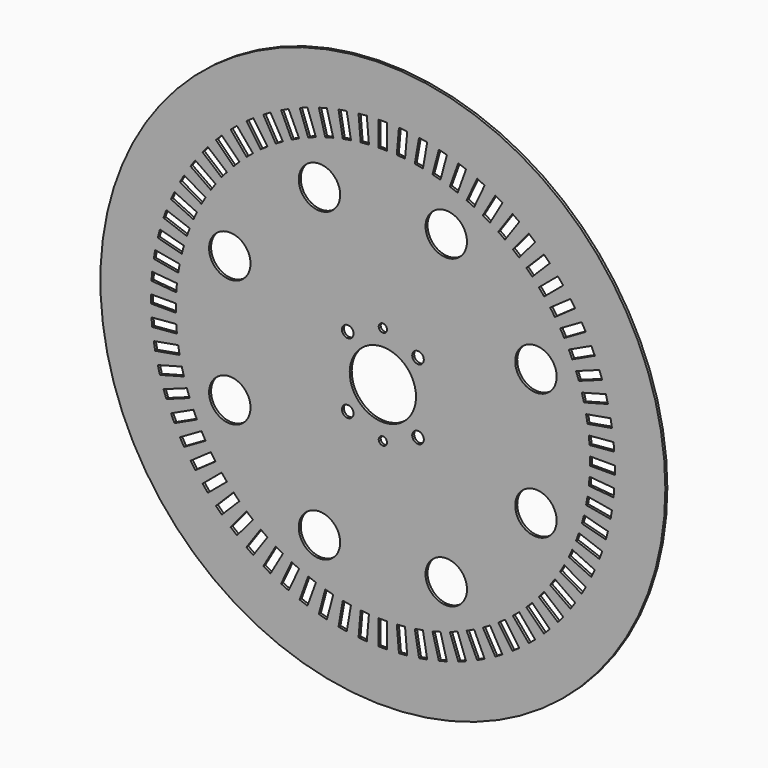
from build123d import *

# Parameters (mm, degrees)
F0_R     = 170.5
F1_DEPTH = 1.5
F3_DEPTH = 25
F5_DEPTH = 25
F7_DEPTH = 25


# Not quite as in the source:
# - ends of sketch curves that miss each other by under 0.0002 mm in the source are joined


with BuildPart() as f1:
    # F0 (on Front) → F1 (new body)
    with BuildSketch(Plane.XZ):
        Circle(F0_R)
        Polygon((-30, 0), (-15, 15), (0, 30), (30, 0), (15, -15), (0, -30), align=None, mode=Mode.SUBTRACT)
        with BuildLine():
            ThreePointArc((-14.1421356237, 14.1421356237), (7.6536686473, 18.4775906502), (20, 0))
            ThreePointArc((20, 0), (18.4775906502, -7.6536686473), (14.1421356237, -14.1421356237))
            Line((14.1421356237, -14.1421356237), (15, -15))
            Line((15, -15), (30, 0))
            Line((30, 0), (0, 30))
            Line((0, 30), (-15, 15))
            Line((-15, 15), (-14.1421356237, 14.1421356237))
        make_face()
        with BuildLine():
            ThreePointArc((14.1421356237, -14.1421356237), (-14.1421356237, -14.1421356237), (-14.1421356237, 14.1421356237))
            Line((-14.1421356237, 14.1421356237), (-15, 15))
            Line((-15, 15), (-30, 0))
            Line((-30, 0), (0, -30))
            Line((0, -30), (15, -15))
            Line((15, -15), (14.1421356237, -14.1421356237))
        make_face()
    extrude(amount=F1_DEPTH)

    # F2 (on face) → F3 (cut)
    with BuildSketch(Plane.XZ.offset(1.5)):
        with BuildLine():
            Line((-17.7132034356, 21.2132034356), (-21.2132034356, 21.2132034356))
            Line((-21.2132034356, 21.2132034356), (-21.2132034356, 17.7132034356))
            ThreePointArc((-21.2132034356, 17.7132034356), (-18.7383297014, 18.7383297014), (-17.7132034356, 21.2132034356))
        make_face()
        with BuildLine():
            ThreePointArc((-23.5394952244, 18.5981763778), (-22.4145176385, 19.9396439044), (-21.2132034356, 21.2132034356))
            ThreePointArc((-21.2132034356, 21.2132034356), (-19.9396439044, 22.4145176385), (-18.5981763778, 23.5394952244))
            ThreePointArc((-18.5981763778, 23.5394952244), (-23.6880771697, 23.6880771697), (-23.5394952244, 18.5981763778))
        make_face()
        with BuildLine():
            Line((-21.2132034356, 17.7132034356), (-21.2132034356, 21.2132034356))
            ThreePointArc((-21.2132034356, 21.2132034356), (-22.4145176385, 19.9396439044), (-23.5394952244, 18.5981763778))
            ThreePointArc((-23.5394952244, 18.5981763778), (-22.4576722575, 17.9419196889), (-21.2132034356, 17.7132034356))
        make_face()
        with BuildLine():
            ThreePointArc((-18.5981763778, 23.5394952244), (-19.9396439044, 22.4145176385), (-21.2132034356, 21.2132034356))
            Line((-21.2132034356, 21.2132034356), (-17.7132034356, 21.2132034356))
            ThreePointArc((-17.7132034356, 21.2132034356), (-17.9419196889, 22.4576722575), (-18.5981763778, 23.5394952244))
        make_face()
        with BuildLine():
            ThreePointArc((-21.2132034356, -21.2132034356), (-22.4145176385, -19.9396439044), (-23.5394952244, -18.5981763778))
            ThreePointArc((-23.5394952244, -18.5981763778), (-23.6880771697, -23.6880771697), (-18.5981763778, -23.5394952244))
            ThreePointArc((-18.5981763778, -23.5394952244), (-19.9396439044, -22.4145176385), (-21.2132034356, -21.2132034356))
        make_face()
        with BuildLine():
            Line((-21.2132034356, -21.2132034356), (-21.2132034356, -17.7132034356))
            ThreePointArc((-21.2132034356, -17.7132034356), (-22.4576722575, -17.9419196889), (-23.5394952244, -18.5981763778))
            ThreePointArc((-23.5394952244, -18.5981763778), (-22.4145176385, -19.9396439044), (-21.2132034356, -21.2132034356))
        make_face()
        with BuildLine():
            ThreePointArc((-17.7132034356, -21.2132034356), (-18.7383297014, -18.7383297014), (-21.2132034356, -17.7132034356))
            Line((-21.2132034356, -17.7132034356), (-21.2132034356, -21.2132034356))
            Line((-21.2132034356, -21.2132034356), (-17.7132034356, -21.2132034356))
        make_face()
        with BuildLine():
            Line((-17.7132034356, -21.2132034356), (-21.2132034356, -21.2132034356))
            ThreePointArc((-21.2132034356, -21.2132034356), (-19.9396439044, -22.4145176385), (-18.5981763778, -23.5394952244))
            ThreePointArc((-18.5981763778, -23.5394952244), (-17.9419196889, -22.4576722575), (-17.7132034356, -21.2132034356))
        make_face()
        with BuildLine():
            ThreePointArc((2.4978289184, -29.8958333333), (0, -27.5), (-2.4978289184, -29.8958333333))
            ThreePointArc((-2.4978289184, -29.8958333333), (0, -30), (2.4978289184, -29.8958333333))
        make_face()
        with BuildLine():
            ThreePointArc((2.4978289184, -29.8958333333), (0, -30), (-2.4978289184, -29.8958333333))
            ThreePointArc((-2.4978289184, -29.8958333333), (-0.0520946447, -32.4994571707), (2.5, -30))
            ThreePointArc((2.5, -30), (2.4994571707, -29.9479053553), (2.4978289184, -29.8958333333))
        make_face()
        with BuildLine():
            ThreePointArc((23.5394952244, -18.5981763778), (22.4145176385, -19.9396439044), (21.2132034356, -21.2132034356))
            ThreePointArc((21.2132034356, -21.2132034356), (19.9396439044, -22.4145176385), (18.5981763778, -23.5394952244))
            ThreePointArc((18.5981763778, -23.5394952244), (22.4576722575, -24.4844871823), (24.7132034356, -21.2132034356))
            ThreePointArc((24.7132034356, -21.2132034356), (24.406322699, -19.7800288581), (23.5394952244, -18.5981763778))
        make_face()
        with BuildLine():
            Line((21.2132034356, -21.2132034356), (21.2132034356, -17.7132034356))
            ThreePointArc((21.2132034356, -17.7132034356), (18.7383297014, -18.7383297014), (17.7132034356, -21.2132034356))
            Line((17.7132034356, -21.2132034356), (21.2132034356, -21.2132034356))
        make_face()
        with BuildLine():
            Line((21.2132034356, -21.2132034356), (17.7132034356, -21.2132034356))
            ThreePointArc((17.7132034356, -21.2132034356), (17.9419196889, -22.4576722575), (18.5981763778, -23.5394952244))
            ThreePointArc((18.5981763778, -23.5394952244), (19.9396439044, -22.4145176385), (21.2132034356, -21.2132034356))
        make_face()
        with BuildLine():
            ThreePointArc((23.5394952244, -18.5981763778), (22.4576722575, -17.9419196889), (21.2132034356, -17.7132034356))
            Line((21.2132034356, -17.7132034356), (21.2132034356, -21.2132034356))
            ThreePointArc((21.2132034356, -21.2132034356), (22.4145176385, -19.9396439044), (23.5394952244, -18.5981763778))
        make_face()
        with BuildLine():
            Line((21.2132034356, 21.2132034356), (17.7132034356, 21.2132034356))
            ThreePointArc((17.7132034356, 21.2132034356), (18.7383297014, 18.7383297014), (21.2132034356, 17.7132034356))
            Line((21.2132034356, 17.7132034356), (21.2132034356, 21.2132034356))
        make_face()
        with BuildLine():
            ThreePointArc((18.5981763778, 23.5394952244), (17.9419196889, 22.4576722575), (17.7132034356, 21.2132034356))
            Line((17.7132034356, 21.2132034356), (21.2132034356, 21.2132034356))
            ThreePointArc((21.2132034356, 21.2132034356), (19.9396439044, 22.4145176385), (18.5981763778, 23.5394952244))
        make_face()
        with BuildLine():
            ThreePointArc((23.5394952244, 18.5981763778), (22.4145176385, 19.9396439044), (21.2132034356, 21.2132034356))
            Line((21.2132034356, 21.2132034356), (21.2132034356, 17.7132034356))
            ThreePointArc((21.2132034356, 17.7132034356), (22.4576722575, 17.9419196889), (23.5394952244, 18.5981763778))
        make_face()
        with BuildLine():
            ThreePointArc((18.5981763778, 23.5394952244), (19.9396439044, 22.4145176385), (21.2132034356, 21.2132034356))
            ThreePointArc((21.2132034356, 21.2132034356), (22.4145176385, 19.9396439044), (23.5394952244, 18.5981763778))
            ThreePointArc((23.5394952244, 18.5981763778), (24.406322699, 19.7800288581), (24.7132034356, 21.2132034356))
            ThreePointArc((24.7132034356, 21.2132034356), (22.4576722575, 24.4844871823), (18.5981763778, 23.5394952244))
        make_face()
        with BuildLine():
            ThreePointArc((2.4978289184, 29.8958333333), (0, 30), (-2.4978289184, 29.8958333333))
            ThreePointArc((-2.4978289184, 29.8958333333), (0, 27.5), (2.4978289184, 29.8958333333))
        make_face()
        with BuildLine():
            ThreePointArc((2.5, 30), (-0.0520946447, 32.4994571707), (-2.4978289184, 29.8958333333))
            ThreePointArc((-2.4978289184, 29.8958333333), (0, 30), (2.4978289184, 29.8958333333))
            ThreePointArc((2.4978289184, 29.8958333333), (2.4994571707, 29.9479053553), (2.5, 30))
        make_face()
    extrude(amount=-F3_DEPTH, mode=Mode.SUBTRACT)

    # F4 (on face) → F5 (cut)
    with BuildSketch(Plane.XZ.offset(1.5)):
        with BuildLine():
            Line((-92.3879532511, 38.2683432365), (-92.3879532511, 25.7683432365))
            ThreePointArc((-92.3879532511, 25.7683432365), (-83.5491184863, 29.4295084717), (-79.8879532511, 38.2683432365))
            ThreePointArc((-79.8879532511, 38.2683432365), (-80.8394590947, 43.0518861411), (-83.5491184863, 47.1071780013))
            Line((-83.5491184863, 47.1071780013), (-92.3879532511, 38.2683432365))
        make_face()
        with BuildLine():
            ThreePointArc((-83.5491184863, 47.1071780013), (-103.9364474075, 43.0518861411), (-92.3879532511, 25.7683432365))
            Line((-92.3879532511, 25.7683432365), (-92.3879532511, 38.2683432365))
            Line((-92.3879532511, 38.2683432365), (-83.5491184863, 47.1071780013))
        make_face()
        with BuildLine():
            Line((-92.3879532511, -38.2683432365), (-83.5491184863, -47.1071780013))
            ThreePointArc((-83.5491184863, -47.1071780013), (-80.8394590947, -43.0518861411), (-79.8879532511, -38.2683432365))
            ThreePointArc((-79.8879532511, -38.2683432365), (-83.5491184863, -29.4295084717), (-92.3879532511, -25.7683432365))
            Line((-92.3879532511, -25.7683432365), (-92.3879532511, -38.2683432365))
        make_face()
        with BuildLine():
            ThreePointArc((-92.3879532511, -25.7683432365), (-103.9364474075, -43.0518861411), (-83.5491184863, -47.1071780013))
            Line((-83.5491184863, -47.1071780013), (-92.3879532511, -38.2683432365))
            Line((-92.3879532511, -38.2683432365), (-92.3879532511, -25.7683432365))
        make_face()
        with BuildLine():
            Line((-38.2683432365, -92.3879532511), (-25.7683432365, -92.3879532511))
            ThreePointArc((-25.7683432365, -92.3879532511), (-33.4848003319, -80.8394590947), (-47.1071780013, -83.5491184863))
            Line((-47.1071780013, -83.5491184863), (-38.2683432365, -92.3879532511))
        make_face()
        with BuildLine():
            ThreePointArc((-47.1071780013, -83.5491184863), (-43.0518861411, -103.9364474075), (-25.7683432365, -92.3879532511))
            Line((-25.7683432365, -92.3879532511), (-38.2683432365, -92.3879532511))
            Line((-38.2683432365, -92.3879532511), (-47.1071780013, -83.5491184863))
        make_face()
        with BuildLine():
            ThreePointArc((47.1071780013, -83.5491184863), (33.4848003319, -80.8394590947), (25.7683432365, -92.3879532511))
            Line((25.7683432365, -92.3879532511), (38.2683432365, -92.3879532511))
            Line((38.2683432365, -92.3879532511), (47.1071780013, -83.5491184863))
        make_face()
        with BuildLine():
            Line((38.2683432365, -92.3879532511), (25.7683432365, -92.3879532511))
            ThreePointArc((25.7683432365, -92.3879532511), (38.2683432365, -104.8879532511), (50.7683432365, -92.3879532511))
            ThreePointArc((50.7683432365, -92.3879532511), (49.8168373929, -87.6044103466), (47.1071780013, -83.5491184863))
            Line((47.1071780013, -83.5491184863), (38.2683432365, -92.3879532511))
        make_face()
        with BuildLine():
            ThreePointArc((92.3879532511, -25.7683432365), (80.8394590947, -33.4848003319), (83.5491184863, -47.1071780013))
            Line((83.5491184863, -47.1071780013), (92.3879532511, -38.2683432365))
            Line((92.3879532511, -38.2683432365), (92.3879532511, -25.7683432365))
        make_face()
        with BuildLine():
            Line((92.3879532511, -38.2683432365), (83.5491184863, -47.1071780013))
            ThreePointArc((83.5491184863, -47.1071780013), (97.1714961557, -49.8168373929), (104.8879532511, -38.2683432365))
            ThreePointArc((104.8879532511, -38.2683432365), (101.226788016, -29.4295084717), (92.3879532511, -25.7683432365))
            Line((92.3879532511, -25.7683432365), (92.3879532511, -38.2683432365))
        make_face()
        with BuildLine():
            ThreePointArc((83.5491184863, 47.1071780013), (80.8394590947, 33.4848003319), (92.3879532511, 25.7683432365))
            Line((92.3879532511, 25.7683432365), (92.3879532511, 38.2683432365))
            Line((92.3879532511, 38.2683432365), (83.5491184863, 47.1071780013))
        make_face()
        with BuildLine():
            Line((92.3879532511, 38.2683432365), (92.3879532511, 25.7683432365))
            ThreePointArc((92.3879532511, 25.7683432365), (101.226788016, 29.4295084717), (104.8879532511, 38.2683432365))
            ThreePointArc((104.8879532511, 38.2683432365), (97.1714961557, 49.8168373929), (83.5491184863, 47.1071780013))
            Line((83.5491184863, 47.1071780013), (92.3879532511, 38.2683432365))
        make_face()
        with BuildLine():
            ThreePointArc((25.7683432365, 92.3879532511), (33.4848003319, 80.8394590947), (47.1071780013, 83.5491184863))
            Line((47.1071780013, 83.5491184863), (38.2683432365, 92.3879532511))
            Line((38.2683432365, 92.3879532511), (25.7683432365, 92.3879532511))
        make_face()
        with BuildLine():
            Line((38.2683432365, 92.3879532511), (47.1071780013, 83.5491184863))
            ThreePointArc((47.1071780013, 83.5491184863), (49.8168373929, 87.6044103466), (50.7683432365, 92.3879532511))
            ThreePointArc((50.7683432365, 92.3879532511), (38.2683432365, 104.8879532511), (25.7683432365, 92.3879532511))
            Line((25.7683432365, 92.3879532511), (38.2683432365, 92.3879532511))
        make_face()
        with BuildLine():
            Line((-38.2683432365, 92.3879532511), (-47.1071780013, 83.5491184863))
            ThreePointArc((-47.1071780013, 83.5491184863), (-33.4848003319, 80.8394590947), (-25.7683432365, 92.3879532511))
            Line((-25.7683432365, 92.3879532511), (-38.2683432365, 92.3879532511))
        make_face()
        with BuildLine():
            ThreePointArc((-25.7683432365, 92.3879532511), (-43.0518861411, 103.9364474075), (-47.1071780013, 83.5491184863))
            Line((-47.1071780013, 83.5491184863), (-38.2683432365, 92.3879532511))
            Line((-38.2683432365, 92.3879532511), (-25.7683432365, 92.3879532511))
        make_face()
    extrude(amount=-F5_DEPTH, mode=Mode.SUBTRACT)

    # F6 (on face) → F7 (cut)
    with BuildSketch(Plane.XZ.offset(1.5)):
        with BuildLine():
            ThreePointArc((-2.49999995, 124.9749975005), (-6.24891e-05, 125), (2.4998749969, 124.975))
            Line((2.4998749969, 124.975), (2.4998749969, 139.975))
            Line((2.4998749969, 139.975), (-2.5, 139.975))
            Line((-2.5, 139.975), (-2.49999995, 124.9749975005))
        make_face()
        with BuildLine():
            ThreePointArc((8.4018020366, 124.7173192565), (10.8944055922, 124.5243427077), (13.3826511677, 124.2815539319))
            Line((13.3826511677, 124.2815539319), (14.6899873089, 139.2244744033))
            Line((14.6899873089, 139.2244744033), (9.7091383459, 139.6602422223))
            Line((9.7091383459, 139.6602422223), (8.4018020366, 124.7173192565))
        make_face()
        with BuildLine():
            ThreePointArc((19.2396612366, 123.5104669067), (21.7059606687, 123.1009799776), (24.1635772824, 122.6422501951))
            Line((24.1635772824, 122.6422501951), (26.7682999474, 137.4143664903))
            Line((26.7682999474, 137.4143664903), (21.8443842864, 138.2825856721))
            Line((21.8443842864, 138.2825856721), (19.2396612366, 123.5104669067))
        make_face()
        with BuildLine():
            ThreePointArc((29.9310949973, 121.363625326), (32.352320278, 120.7407444595), (34.7606039837, 120.0695648809))
            Line((34.7606039837, 120.0695648809), (38.6428896602, 134.5584522752))
            Line((38.6428896602, 134.5584522752), (33.8133812725, 135.8525151476))
            Line((33.8133812725, 135.8525151476), (29.9310949973, 121.363625326))
        make_face()
        with BuildLine():
            ThreePointArc((40.3947350523, 118.2931332752), (42.7524591952, 117.4615989707), (45.0930814996, 116.583077678))
            Line((45.0930814996, 116.583077678), (50.2233836495, 130.6784669898))
            Line((50.2233836495, 130.6784669898), (45.52503801, 132.3885249528))
            Line((45.52503801, 132.3885249528), (40.3947350523, 118.2931332752))
        make_face()
        with BuildLine():
            ThreePointArc((50.5509467824, 114.3223590528), (52.8272260833, 113.2884997886), (55.0823734373, 112.2093228592))
            Line((55.0823734373, 112.2093228592), (61.4216473634, 125.8039396647))
            Line((61.4216473634, 125.8039396647), (56.8902217196, 127.9169781448))
            Line((56.8902217196, 127.9169781448), (50.5509467824, 114.3223590528))
        make_face()
        with BuildLine():
            ThreePointArc((60.3224352841, 109.4815226483), (62.4999458829, 108.2532067176), (64.6524552536, 106.9815873395))
            Line((64.6524552536, 106.9815873395), (72.1524552536, 119.9719683963))
            Line((72.1524552536, 119.9719683963), (67.8224364905, 122.4719058947))
            Line((67.8224364905, 122.4719058947), (60.3224352841, 109.4815226483))
        make_face()
        with BuildLine():
            ThreePointArc((69.6348336296, 103.8074657497), (71.6970033558, 102.3940413784), (73.7304928471, 100.939657343))
            Line((73.7304928471, 100.939657343), (82.3341393924, 113.2269380073))
            Line((82.3341393924, 113.2269380073), (78.2384815675, 116.0947484902))
            Line((78.2384815675, 116.0947484902), (69.6348336296, 103.8074657497))
        make_face()
        with BuildLine():
            ThreePointArc((78.4172688444, 97.3433713561), (80.3484033414, 95.7555955571), (82.2473968704, 94.129515605))
            Line((82.2473968704, 94.129515605), (91.8892110157, 105.6201822518))
            Line((91.8892110157, 105.6201822518), (88.0590845581, 108.8340399498))
            Line((88.0590845581, 108.8340399498), (78.4172688444, 97.3433713561))
        make_face()
        with BuildLine():
            ThreePointArc((86.6029012938, 90.138435129), (88.3883034619, 88.3883918347), (90.1383485412, 86.6029914164))
            Line((90.1383485412, 86.6029914164), (100.744950259, 97.2095931342))
            Line((100.744950259, 97.2095931342), (97.2095047436, 100.7450386496))
            Line((97.2095047436, 100.7450386496), (86.6029012938, 90.138435129))
        make_face()
        with BuildLine():
            ThreePointArc((94.129433372, 82.2474909834), (95.7555152227, 80.3484990802), (97.3432929526, 78.4173661707))
            Line((97.3432929526, 78.4173661707), (108.8339595993, 88.059180316))
            Line((108.8339595993, 88.059180316), (105.6201019014, 91.8893067737))
            Line((105.6201019014, 91.8893067737), (94.129433372, 82.2474909834))
        make_face()
        with BuildLine():
            ThreePointArc((100.9395836253, 73.7305937691), (102.3939696939, 71.6971057319), (103.807396127, 69.6349374188))
            Line((103.807396127, 69.6349374188), (116.0946767914, 78.2385839641))
            Line((116.0946767914, 78.2385839641), (113.2268663085, 82.334241789))
            Line((113.2268663085, 82.334241789), (100.9395836253, 73.7305937691))
        make_face()
        with BuildLine():
            ThreePointArc((106.9815226983, 64.6525622164), (108.2531442285, 62.5000541171), (109.4814623364, 60.3225447464))
            Line((109.4814623364, 60.3225447464), (122.4718433932, 67.8225447464))
            Line((122.4718433932, 67.8225447464), (119.9719058947, 72.1525635095))
            Line((119.9719058947, 72.1525635095), (106.9815226983, 64.6525622164))
        make_face()
        with BuildLine():
            ThreePointArc((112.2092677864, 55.082485627), (113.2884469705, 52.8273393519), (114.3223085107, 50.5510610848))
            Line((114.3223085107, 50.5510610848), (127.9169253162, 56.8903350109))
            Line((127.9169253162, 56.8903350109), (125.8038868361, 61.4217606547))
            Line((125.8038868361, 61.4217606547), (112.2092677864, 55.082485627))
        make_face()
        with BuildLine():
            ThreePointArc((116.5830325927, 45.0931980622), (117.4615562257, 42.7525766362), (118.2930928874, 40.3948533247))
            Line((118.2930928874, 40.3948533247), (132.3884821992, 45.5251554746))
            Line((132.3884821992, 45.5251554746), (130.6784242362, 50.223501114))
            Line((130.6784242362, 50.223501114), (116.5830325927, 45.0931980622))
        make_face()
        with BuildLine():
            ThreePointArc((120.0695301263, 34.7607240322), (120.7407121128, 32.3524409976), (121.3635954, 29.9312163397))
            Line((121.3635954, 29.9312163397), (135.8524827944, 33.8135020162))
            Line((135.8524827944, 33.8135020162), (134.5584199221, 38.6430104039))
            Line((134.5584199221, 38.6430104039), (120.0695301263, 34.7607240322))
        make_face()
        with BuildLine():
            ThreePointArc((122.6422260357, 24.1636999032), (123.1009582754, 21.7060837481), (123.5104476703, 19.2397847254))
            Line((123.5104476703, 19.2397847254), (138.2825639655, 21.8445073904))
            Line((138.2825639655, 21.8445073904), (137.4143447837, 26.7684230515))
            Line((137.4143447837, 26.7684230515), (122.6422260357, 24.1636999032))
        make_face()
        with BuildLine():
            ThreePointArc((124.2815405515, 13.3827754275), (124.5243318152, 10.8945300947), (124.7173108561, 8.4019267321))
            Line((124.7173108561, 8.4019267321), (139.6602313275, 9.7092628733))
            Line((139.6602313275, 9.7092628733), (139.2244635085, 14.6901118363))
            Line((139.2244635085, 14.6901118363), (124.2815405515, 13.3827754275))
        make_face()
        with BuildLine():
            ThreePointArc((124.9749975005, 2.49999995), (124.9937492188, 1.2500624859), (125, 0))
            ThreePointArc((125, 0), (124.9937498437, -1.25), (124.975, -2.4998749969))
            Line((124.975, -2.4998749969), (139.975, -2.4998749969))
            Line((139.975, -2.4998749969), (139.975, 2.5))
            Line((139.975, 2.5), (124.9749975005, 2.49999995))
        make_face()
        with BuildLine():
            Line((139.6602422223, -9.7091383459), (124.7173217509, -8.4018022047))
            ThreePointArc((124.7173217509, -8.4018022047), (124.5243427077, -10.8944055922), (124.2815539319, -13.3826511677))
            Line((124.2815539319, -13.3826511677), (139.2244744033, -14.6899873089))
            Line((139.2244744033, -14.6899873089), (139.6602422223, -9.7091383459))
        make_face()
        with BuildLine():
            Line((138.2825856721, -21.8443842864), (123.5104693769, -19.2396616214))
            ThreePointArc((123.5104693769, -19.2396616214), (123.1009799776, -21.7059606687), (122.6422501951, -24.1635772824))
            Line((122.6422501951, -24.1635772824), (137.4143664903, -26.7682999474))
            Line((137.4143664903, -26.7682999474), (138.2825856721, -21.8443842864))
        make_face()
        with BuildLine():
            Line((135.8525151476, -33.8133812725), (121.3636277532, -29.931095596))
            ThreePointArc((121.3636277532, -29.931095596), (120.7407444595, -32.352320278), (120.0695648809, -34.7606039837))
            Line((120.0695648809, -34.7606039837), (134.5584522752, -38.6428896602))
            Line((134.5584522752, -38.6428896602), (135.8525151476, -33.8133812725))
        make_face()
        with BuildLine():
            Line((127.9169781448, -56.8902217196), (114.3223613393, -50.5509477935))
            ThreePointArc((114.3223613393, -50.5509477935), (113.2884997886, -52.8272260833), (112.2093228592, -55.0823734373))
            Line((112.2093228592, -55.0823734373), (125.8039396647, -61.4216473634))
            Line((125.8039396647, -61.4216473634), (127.9169781448, -56.8902217196))
        make_face()
        with BuildLine():
            Line((132.3885249528, -45.52503801), (118.293135641, -40.3947358602))
            ThreePointArc((118.293135641, -40.3947358602), (117.4615989707, -42.7524591952), (116.583077678, -45.0930814996))
            Line((116.583077678, -45.0930814996), (130.6784669898, -50.2233836495))
            Line((130.6784669898, -50.2233836495), (132.3885249528, -45.52503801))
        make_face()
        with BuildLine():
            Line((122.4719058947, -67.8224364905), (109.481524838, -60.3224364905))
            ThreePointArc((109.481524838, -60.3224364905), (108.2532067176, -62.4999458829), (106.9815873395, -64.6524552536))
            Line((106.9815873395, -64.6524552536), (119.9719683963, -72.1524552536))
            Line((119.9719683963, -72.1524552536), (122.4719058947, -67.8224364905))
        make_face()
        with BuildLine():
            Line((116.0947484902, -78.2384815675), (103.8074678259, -69.6348350222))
            ThreePointArc((103.8074678259, -69.6348350222), (102.3940413784, -71.6970033558), (100.939657343, -73.7304928471))
            Line((100.939657343, -73.7304928471), (113.2269380073, -82.3341393924))
            Line((113.2269380073, -82.3341393924), (116.0947484902, -78.2384815675))
        make_face()
        with BuildLine():
            Line((108.8340399498, -88.0590845581), (97.343373303, -78.4172704128))
            ThreePointArc((97.343373303, -78.4172704128), (95.7555955571, -80.3484033414), (94.129515605, -82.2473968704))
            Line((94.129515605, -82.2473968704), (105.6201822518, -91.8892110157))
            Line((105.6201822518, -91.8892110157), (108.8340399498, -88.0590845581))
        make_face()
        with BuildLine():
            Line((100.7450386496, -97.2095047436), (90.1384369318, -86.6029030258))
            ThreePointArc((90.1384369318, -86.6029030258), (88.3883918347, -88.3883034619), (86.6029914164, -90.1383485412))
            Line((86.6029914164, -90.1383485412), (97.2095931342, -100.744950259))
            Line((97.2095931342, -100.744950259), (100.7450386496, -97.2095047436))
        make_face()
        with BuildLine():
            Line((91.8893067737, -105.6201019014), (82.2474926284, -94.1294352546))
            ThreePointArc((82.2474926284, -94.1294352546), (80.3484990802, -95.7555152227), (78.4173661707, -97.3432929526))
            Line((78.4173661707, -97.3432929526), (88.059180316, -108.8339595993))
            Line((88.059180316, -108.8339595993), (91.8893067737, -105.6201019014))
        make_face()
        with BuildLine():
            Line((82.334241789, -113.2268663085), (73.7305952437, -100.9395856441))
            ThreePointArc((73.7305952437, -100.9395856441), (71.6971057319, -102.3939696939), (69.6349374188, -103.807396127))
            Line((69.6349374188, -103.807396127), (78.2385839641, -116.0946767914))
            Line((78.2385839641, -116.0946767914), (82.334241789, -113.2268663085))
        make_face()
        with BuildLine():
            Line((72.1525635095, -119.9719058947), (64.6525635095, -106.981524838))
            ThreePointArc((64.6525635095, -106.981524838), (62.5000541171, -108.2531442285), (60.3225447464, -109.4814623364))
            Line((60.3225447464, -109.4814623364), (67.8225447464, -122.4718433932))
            Line((67.8225447464, -122.4718433932), (72.1525635095, -119.9719058947))
        make_face()
        with BuildLine():
            Line((50.223501114, -130.6784242362), (45.0931989641, -116.5830349244))
            ThreePointArc((45.0931989641, -116.5830349244), (42.7525766362, -117.4615562257), (40.3948533247, -118.2930928874))
            Line((40.3948533247, -118.2930928874), (45.5251554746, -132.3884821992))
            Line((45.5251554746, -132.3884821992), (50.223501114, -130.6784242362))
        make_face()
        with BuildLine():
            Line((38.6430104039, -134.5584199221), (34.7607247274, -120.0695325277))
            ThreePointArc((34.7607247274, -120.0695325277), (32.3524409976, -120.7407121128), (29.9312163397, -121.3635954))
            Line((29.9312163397, -121.3635954), (33.8135020162, -135.8524827944))
            Line((33.8135020162, -135.8524827944), (38.6430104039, -134.5584199221))
        make_face()
        with BuildLine():
            Line((26.7684230515, -137.4143447837), (24.1637003865, -122.6422284885))
            ThreePointArc((24.1637003865, -122.6422284885), (21.7060837481, -123.1009582754), (19.2397847254, -123.5104476703))
            Line((19.2397847254, -123.5104476703), (21.8445073904, -138.2825639655))
            Line((21.8445073904, -138.2825639655), (26.7684230515, -137.4143447837))
        make_face()
        with BuildLine():
            Line((14.6901118363, -139.2244635085), (13.3827756951, -124.2815430371))
            ThreePointArc((13.3827756951, -124.2815430371), (10.8945300947, -124.5243318152), (8.4019267321, -124.7173108561))
            Line((8.4019267321, -124.7173108561), (9.7092628733, -139.6602313275))
            Line((9.7092628733, -139.6602313275), (14.6901118363, -139.2244635085))
        make_face()
        with BuildLine():
            Line((2.5, -139.975), (2.5, -124.975))
            ThreePointArc((2.5, -124.975), (6.24891e-05, -125), (-2.4998749969, -124.975))
            Line((-2.4998749969, -124.975), (-2.4998749969, -139.975))
            Line((-2.4998749969, -139.975), (2.5, -139.975))
        make_face()
        with BuildLine():
            Line((-9.7091383459, -139.6602422223), (-8.4018022047, -124.7173217509))
            ThreePointArc((-8.4018022047, -124.7173217509), (-10.8944055922, -124.5243427077), (-13.3826511677, -124.2815539319))
            Line((-13.3826511677, -124.2815539319), (-14.6899873089, -139.2244744033))
            Line((-14.6899873089, -139.2244744033), (-9.7091383459, -139.6602422223))
        make_face()
        with BuildLine():
            Line((-21.8443842864, -138.2825856721), (-19.2396616214, -123.5104693769))
            ThreePointArc((-19.2396616214, -123.5104693769), (-21.7059606687, -123.1009799776), (-24.1635772824, -122.6422501951))
            Line((-24.1635772824, -122.6422501951), (-26.7682999474, -137.4143664903))
            Line((-26.7682999474, -137.4143664903), (-21.8443842864, -138.2825856721))
        make_face()
        with BuildLine():
            Line((61.4217606547, -125.8038868361), (55.0824867286, -112.2092700306))
            ThreePointArc((55.0824867286, -112.2092700306), (52.8273393519, -113.2884469705), (50.5510610848, -114.3223085107))
            Line((50.5510610848, -114.3223085107), (56.8903350109, -127.9169253162))
            Line((56.8903350109, -127.9169253162), (61.4217606547, -125.8038868361))
        make_face()
        with BuildLine():
            Line((-33.8133812725, -135.8525151476), (-29.931095596, -121.3636277532))
            ThreePointArc((-29.931095596, -121.3636277532), (-32.352320278, -120.7407444595), (-34.7606039837, -120.0695648809))
            Line((-34.7606039837, -120.0695648809), (-38.6428896602, -134.5584522752))
            Line((-38.6428896602, -134.5584522752), (-33.8133812725, -135.8525151476))
        make_face()
        with BuildLine():
            Line((-45.52503801, -132.3885249528), (-40.3947358602, -118.293135641))
            ThreePointArc((-40.3947358602, -118.293135641), (-42.7524591952, -117.4615989707), (-45.0930814996, -116.583077678))
            Line((-45.0930814996, -116.583077678), (-50.2233836495, -130.6784669898))
            Line((-50.2233836495, -130.6784669898), (-45.52503801, -132.3885249528))
        make_face()
        with BuildLine():
            Line((-56.8902217196, -127.9169781448), (-50.5509477935, -114.3223613393))
            ThreePointArc((-50.5509477935, -114.3223613393), (-52.8272260833, -113.2884997886), (-55.0823734373, -112.2093228592))
            Line((-55.0823734373, -112.2093228592), (-61.4216473634, -125.8039396647))
            Line((-61.4216473634, -125.8039396647), (-56.8902217196, -127.9169781448))
        make_face()
        with BuildLine():
            Line((-67.8224364905, -122.4719058947), (-60.3224364905, -109.481524838))
            ThreePointArc((-60.3224364905, -109.481524838), (-62.4999458829, -108.2532067176), (-64.6524552536, -106.9815873395))
            Line((-64.6524552536, -106.9815873395), (-72.1524552536, -119.9719683963))
            Line((-72.1524552536, -119.9719683963), (-67.8224364905, -122.4719058947))
        make_face()
        with BuildLine():
            Line((-78.2384815675, -116.0947484902), (-69.6348350222, -103.8074678259))
            ThreePointArc((-69.6348350222, -103.8074678259), (-71.6970033558, -102.3940413784), (-73.7304928471, -100.939657343))
            Line((-73.7304928471, -100.939657343), (-82.3341393924, -113.2269380073))
            Line((-82.3341393924, -113.2269380073), (-78.2384815675, -116.0947484902))
        make_face()
        with BuildLine():
            Line((-88.0590845581, -108.8340399498), (-78.4172704128, -97.343373303))
            ThreePointArc((-78.4172704128, -97.343373303), (-80.3484033414, -95.7555955571), (-82.2473968704, -94.129515605))
            Line((-82.2473968704, -94.129515605), (-91.8892110157, -105.6201822518))
            Line((-91.8892110157, -105.6201822518), (-88.0590845581, -108.8340399498))
        make_face()
        with BuildLine():
            Line((-97.2095047436, -100.7450386496), (-86.6029030258, -90.1384369318))
            ThreePointArc((-86.6029030258, -90.1384369318), (-88.3883034619, -88.3883918347), (-90.1383485412, -86.6029914164))
            Line((-90.1383485412, -86.6029914164), (-100.744950259, -97.2095931342))
            Line((-100.744950259, -97.2095931342), (-97.2095047436, -100.7450386496))
        make_face()
        with BuildLine():
            Line((-105.6201019014, -91.8893067737), (-94.1294352546, -82.2474926284))
            ThreePointArc((-94.1294352546, -82.2474926284), (-95.7555152227, -80.3484990802), (-97.3432929526, -78.4173661707))
            Line((-97.3432929526, -78.4173661707), (-108.8339595993, -88.059180316))
            Line((-108.8339595993, -88.059180316), (-105.6201019014, -91.8893067737))
        make_face()
        with BuildLine():
            Line((-119.9719058947, -72.1525635095), (-106.981524838, -64.6525635095))
            ThreePointArc((-106.981524838, -64.6525635095), (-108.2531442285, -62.5000541171), (-109.4814623364, -60.3225447464))
            Line((-109.4814623364, -60.3225447464), (-122.4718433932, -67.8225447464))
            Line((-122.4718433932, -67.8225447464), (-119.9719058947, -72.1525635095))
        make_face()
        with BuildLine():
            Line((-125.8038868361, -61.4217606547), (-112.2092700306, -55.0824867286))
            ThreePointArc((-112.2092700306, -55.0824867286), (-113.2884469705, -52.8273393519), (-114.3223085107, -50.5510610848))
            Line((-114.3223085107, -50.5510610848), (-127.9169253162, -56.8903350109))
            Line((-127.9169253162, -56.8903350109), (-125.8038868361, -61.4217606547))
        make_face()
        with BuildLine():
            Line((-113.2268663085, -82.334241789), (-100.9395856441, -73.7305952437))
            ThreePointArc((-100.9395856441, -73.7305952437), (-102.3939696939, -71.6971057319), (-103.807396127, -69.6349374188))
            Line((-103.807396127, -69.6349374188), (-116.0946767914, -78.2385839641))
            Line((-116.0946767914, -78.2385839641), (-113.2268663085, -82.334241789))
        make_face()
        with BuildLine():
            Line((-130.6784242362, -50.223501114), (-116.5830349244, -45.0931989641))
            ThreePointArc((-116.5830349244, -45.0931989641), (-117.4615562257, -42.7525766362), (-118.2930928874, -40.3948533247))
            Line((-118.2930928874, -40.3948533247), (-132.3884821992, -45.5251554746))
            Line((-132.3884821992, -45.5251554746), (-130.6784242362, -50.223501114))
        make_face()
        with BuildLine():
            Line((-134.5584199221, -38.6430104039), (-120.0695325277, -34.7607247274))
            ThreePointArc((-120.0695325277, -34.7607247274), (-120.7407121128, -32.3524409976), (-121.3635954, -29.9312163397))
            Line((-121.3635954, -29.9312163397), (-135.8524827944, -33.8135020162))
            Line((-135.8524827944, -33.8135020162), (-134.5584199221, -38.6430104039))
        make_face()
        with BuildLine():
            Line((-137.4143447837, -26.7684230515), (-122.6422284885, -24.1637003865))
            ThreePointArc((-122.6422284885, -24.1637003865), (-123.1009582754, -21.7060837481), (-123.5104476703, -19.2397847254))
            Line((-123.5104476703, -19.2397847254), (-138.2825639655, -21.8445073904))
            Line((-138.2825639655, -21.8445073904), (-137.4143447837, -26.7684230515))
        make_face()
        with BuildLine():
            Line((-139.2244635085, -14.6901118363), (-124.2815430371, -13.3827756951))
            ThreePointArc((-124.2815430371, -13.3827756951), (-124.5243318152, -10.8945300947), (-124.7173108561, -8.4019267321))
            Line((-124.7173108561, -8.4019267321), (-139.6602313275, -9.7092628733))
            Line((-139.6602313275, -9.7092628733), (-139.2244635085, -14.6901118363))
        make_face()
        with BuildLine():
            ThreePointArc((-124.9749975005, -2.49999995), (-125, -6.24891e-05), (-124.975, 2.4998749969))
            Line((-124.975, 2.4998749969), (-139.975, 2.4998749969))
            Line((-139.975, 2.4998749969), (-139.975, -2.5))
            Line((-139.975, -2.5), (-124.9749975005, -2.49999995))
        make_face()
        with BuildLine():
            ThreePointArc((-124.7173192565, 8.4018020366), (-124.5243427077, 10.8944055922), (-124.2815539319, 13.3826511677))
            Line((-124.2815539319, 13.3826511677), (-139.2244744033, 14.6899873089))
            Line((-139.2244744033, 14.6899873089), (-139.6602422223, 9.7091383459))
            Line((-139.6602422223, 9.7091383459), (-124.7173192565, 8.4018020366))
        make_face()
        with BuildLine():
            ThreePointArc((-123.5104669067, 19.2396612366), (-123.1009799776, 21.7059606687), (-122.6422501951, 24.1635772824))
            Line((-122.6422501951, 24.1635772824), (-137.4143664903, 26.7682999474))
            Line((-137.4143664903, 26.7682999474), (-138.2825856721, 21.8443842864))
            Line((-138.2825856721, 21.8443842864), (-123.5104669067, 19.2396612366))
        make_face()
        with BuildLine():
            ThreePointArc((-118.2931332752, 40.3947350523), (-117.4615989707, 42.7524591952), (-116.583077678, 45.0930814996))
            Line((-116.583077678, 45.0930814996), (-130.6784669898, 50.2233836495))
            Line((-130.6784669898, 50.2233836495), (-132.3885249528, 45.52503801))
            Line((-132.3885249528, 45.52503801), (-118.2931332752, 40.3947350523))
        make_face()
        with BuildLine():
            ThreePointArc((-114.3223590528, 50.5509467824), (-113.2884997886, 52.8272260833), (-112.2093228592, 55.0823734373))
            Line((-112.2093228592, 55.0823734373), (-125.8039396647, 61.4216473634))
            Line((-125.8039396647, 61.4216473634), (-127.9169781448, 56.8902217196))
            Line((-127.9169781448, 56.8902217196), (-114.3223590528, 50.5509467824))
        make_face()
        with BuildLine():
            ThreePointArc((-109.4815226483, 60.3224352841), (-108.2532067176, 62.4999458829), (-106.9815873395, 64.6524552536))
            Line((-106.9815873395, 64.6524552536), (-119.9719683963, 72.1524552536))
            Line((-119.9719683963, 72.1524552536), (-122.4719058947, 67.8224364905))
            Line((-122.4719058947, 67.8224364905), (-109.4815226483, 60.3224352841))
        make_face()
        with BuildLine():
            ThreePointArc((-13.3827754275, 124.2815405515), (-10.8945300947, 124.5243318152), (-8.4019267321, 124.7173108561))
            Line((-8.4019267321, 124.7173108561), (-9.7092628733, 139.6602313275))
            Line((-9.7092628733, 139.6602313275), (-14.6901118363, 139.2244635085))
            Line((-14.6901118363, 139.2244635085), (-13.3827754275, 124.2815405515))
        make_face()
        with BuildLine():
            ThreePointArc((-24.1636999032, 122.6422260357), (-21.7060837481, 123.1009582754), (-19.2397847254, 123.5104476703))
            Line((-19.2397847254, 123.5104476703), (-21.8445073904, 138.2825639655))
            Line((-21.8445073904, 138.2825639655), (-26.7684230515, 137.4143447837))
            Line((-26.7684230515, 137.4143447837), (-24.1636999032, 122.6422260357))
        make_face()
        with BuildLine():
            ThreePointArc((-45.0931980622, 116.5830325927), (-42.7525766362, 117.4615562257), (-40.3948533247, 118.2930928874))
            Line((-40.3948533247, 118.2930928874), (-45.5251554746, 132.3884821992))
            Line((-45.5251554746, 132.3884821992), (-50.223501114, 130.6784242362))
            Line((-50.223501114, 130.6784242362), (-45.0931980622, 116.5830325927))
        make_face()
        with BuildLine():
            ThreePointArc((-55.082485627, 112.2092677864), (-52.8273393519, 113.2884469705), (-50.5510610848, 114.3223085107))
            Line((-50.5510610848, 114.3223085107), (-56.8903350109, 127.9169253162))
            Line((-56.8903350109, 127.9169253162), (-61.4217606547, 125.8038868361))
            Line((-61.4217606547, 125.8038868361), (-55.082485627, 112.2092677864))
        make_face()
        with BuildLine():
            ThreePointArc((-34.7607240322, 120.0695301263), (-32.3524409976, 120.7407121128), (-29.9312163397, 121.3635954))
            Line((-29.9312163397, 121.3635954), (-33.8135020162, 135.8524827944))
            Line((-33.8135020162, 135.8524827944), (-38.6430104039, 134.5584199221))
            Line((-38.6430104039, 134.5584199221), (-34.7607240322, 120.0695301263))
        make_face()
        with BuildLine():
            ThreePointArc((-64.6525622164, 106.9815226983), (-62.5000541171, 108.2531442285), (-60.3225447464, 109.4814623364))
            Line((-60.3225447464, 109.4814623364), (-67.8225447464, 122.4718433932))
            Line((-67.8225447464, 122.4718433932), (-72.1525635095, 119.9719058947))
            Line((-72.1525635095, 119.9719058947), (-64.6525622164, 106.9815226983))
        make_face()
        with BuildLine():
            ThreePointArc((-73.7305937691, 100.9395836253), (-71.6971057319, 102.3939696939), (-69.6349374188, 103.807396127))
            Line((-69.6349374188, 103.807396127), (-78.2385839641, 116.0946767914))
            Line((-78.2385839641, 116.0946767914), (-82.334241789, 113.2268663085))
            Line((-82.334241789, 113.2268663085), (-73.7305937691, 100.9395836253))
        make_face()
        with BuildLine():
            ThreePointArc((-82.2474909834, 94.129433372), (-80.3484990802, 95.7555152227), (-78.4173661707, 97.3432929526))
            Line((-78.4173661707, 97.3432929526), (-88.059180316, 108.8339595993))
            Line((-88.059180316, 108.8339595993), (-91.8893067737, 105.6201019014))
            Line((-91.8893067737, 105.6201019014), (-82.2474909834, 94.129433372))
        make_face()
        with BuildLine():
            ThreePointArc((-90.138435129, 86.6029012938), (-88.3883918347, 88.3883034619), (-86.6029914164, 90.1383485412))
            Line((-86.6029914164, 90.1383485412), (-97.2095931342, 100.744950259))
            Line((-97.2095931342, 100.744950259), (-100.7450386496, 97.2095047436))
            Line((-100.7450386496, 97.2095047436), (-90.138435129, 86.6029012938))
        make_face()
        with BuildLine():
            ThreePointArc((-97.3433713561, 78.4172688444), (-95.7555955571, 80.3484033414), (-94.129515605, 82.2473968704))
            Line((-94.129515605, 82.2473968704), (-105.6201822518, 91.8892110157))
            Line((-105.6201822518, 91.8892110157), (-108.8340399498, 88.0590845581))
            Line((-108.8340399498, 88.0590845581), (-97.3433713561, 78.4172688444))
        make_face()
        with BuildLine():
            ThreePointArc((-103.8074657497, 69.6348336296), (-102.3940413784, 71.6970033558), (-100.939657343, 73.7304928471))
            Line((-100.939657343, 73.7304928471), (-113.2269380073, 82.3341393924))
            Line((-113.2269380073, 82.3341393924), (-116.0947484902, 78.2384815675))
            Line((-116.0947484902, 78.2384815675), (-103.8074657497, 69.6348336296))
        make_face()
        with BuildLine():
            ThreePointArc((-121.363625326, 29.9310949973), (-120.7407444595, 32.352320278), (-120.0695648809, 34.7606039837))
            Line((-120.0695648809, 34.7606039837), (-134.5584522752, 38.6428896602))
            Line((-134.5584522752, 38.6428896602), (-135.8525151476, 33.8133812725))
            Line((-135.8525151476, 33.8133812725), (-121.363625326, 29.9310949973))
        make_face()
    extrude(amount=-F7_DEPTH, mode=Mode.SUBTRACT)


solid = f1.part
